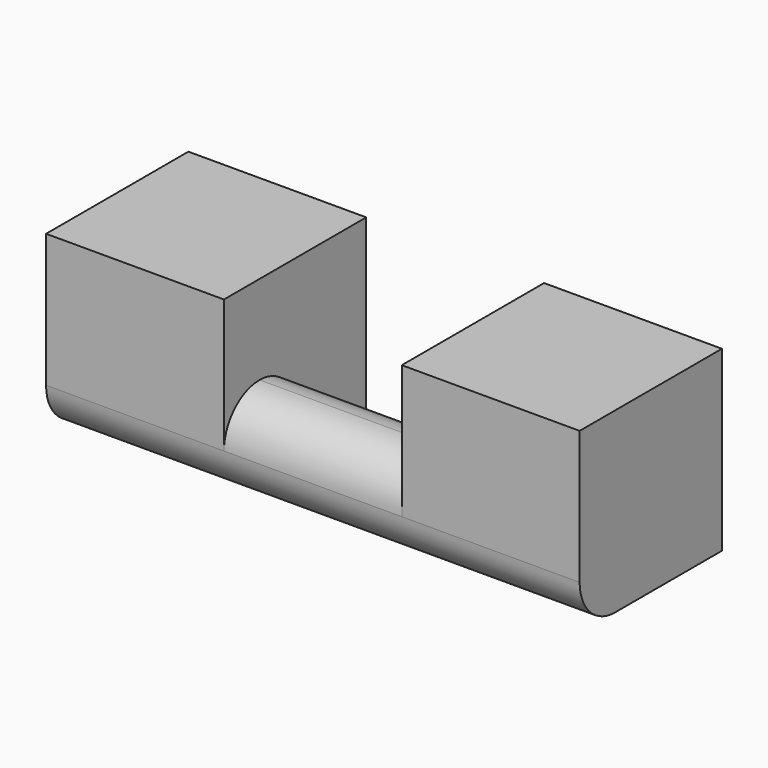
from build123d import *

# Parameters (mm, degrees)
F0_W     = 20
F0_H     = 20
F1_DEPTH = 30
F2_W     = 20
F2_H     = 10
F3_DEPTH = 20
F4_W     = 20
F4_H     = 10
F5_DEPTH = 25
F6_R     = 4.99999


# Not quite as in the source:
# - a fillet or chamfer is up to 0.001 mm smaller than in the source, because OpenCascade refuses the exact size


with BuildPart() as f1:
    # F0 (on Right) → F1 (new body, symmetric)
    with BuildSketch(Plane.YZ):
        Rectangle(F0_W, F0_H)
    extrude(amount=F1_DEPTH, both=True)

    # F2 (on face) → F3 (cut)
    with BuildSketch(Plane.XZ.offset(10)):
        with Locations((0, 5)):
            Rectangle(F2_W, F2_H)
    extrude(amount=-F3_DEPTH, mode=Mode.SUBTRACT)

    # F4 (on face) → F5 (cut)
    with BuildSketch(Plane.XY):
        with Locations((0, 5)):
            Rectangle(F4_W, F4_H)
    extrude(amount=-F5_DEPTH, mode=Mode.SUBTRACT)

    # F6 (radius 5 in the source; OpenCascade refuses exactly that, so slightly less here)
    f6_edges = [f1.edges().sort_by_distance(p)[0] for p in [
        (0, 0, 0),
        (0, 0, -10),
        (0, -10, 0),
        (0, -10, -10),
    ]]
    fillet(f6_edges, radius=F6_R)


solid = f1.part
